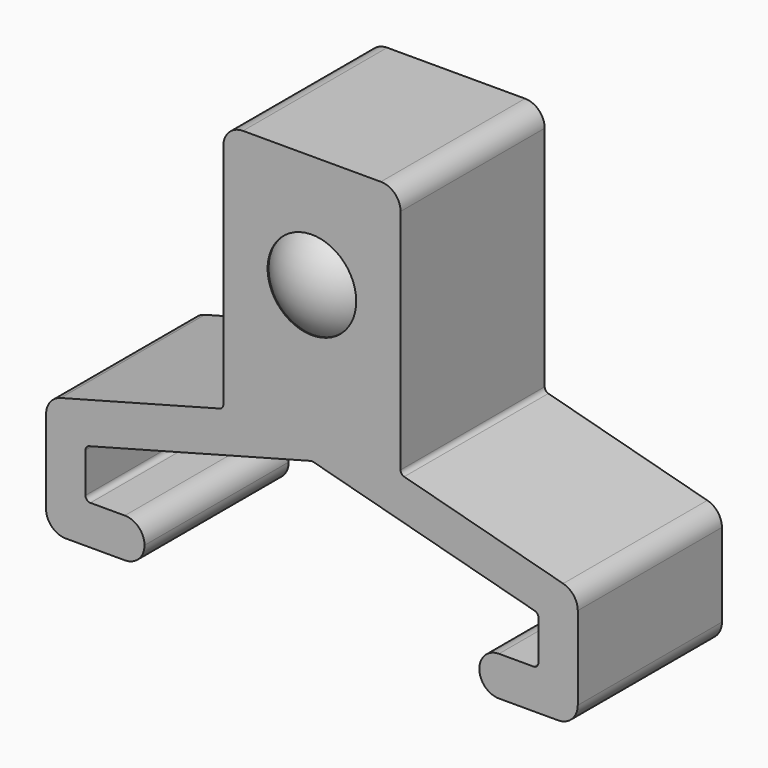
from build123d import *

# Parameters (mm, degrees)
F1_DEPTH      = 4.575
F1_DEPTH_BACK = 4.575
F2_R          = 2.25
F3_DEPTH      = 6
F4_R          = 0.99999
F5_R          = 0.25


# Not quite as in the source:
# - a fillet or chamfer is up to 0.001 mm smaller than in the source, because OpenCascade refuses the exact size


with BuildPart() as f1:
    # F0 (on Front) → F1 (new body, two sides)
    with BuildSketch(Plane.XZ) as f1_sk:
        Polygon((-13.5, 3), (-13.5, -3), (-8.5, -3), (-8.5, -1), (-11.5, -1), (-11.5, 1.4634433738), (0, 4.5301100405), (11.5, 1.4634433738), (11.5, -1), (8.5, -1), (8.5, -3), (13.5, -3), (13.5, 3), (4.5, 5.4), (4.5, 18.15), (-4.5, 18.15), (-4.5, 5.4), align=None)
    extrude(amount=F1_DEPTH)
    extrude(f1_sk.sketch, amount=-F1_DEPTH_BACK)

    # F2 (on face) → F3 (cut)
    with BuildSketch(Plane.XZ.offset(4.575)):
        with Locations((0, 12.4)):
            Circle(F2_R)
    extrude(amount=-F3_DEPTH, mode=Mode.SUBTRACT)

    # F4 (radius 1 in the source; OpenCascade refuses exactly that, so slightly less here)
    f4_edges = [f1.edges().sort_by_distance(p)[0] for p in [
        (-4.5, 0, 18.15),
        (4.5, 0, 18.15),
        (13.5, 0, 3),
        (13.5, 0, -3),
        (8.5, 0, -3),
        (8.5, 0, -1),
        (-8.5, 0, -3),
        (-8.5, 0, -1),
        (-13.5, 0, 3),
        (-13.5, 0, -3),
    ]]
    fillet(f4_edges, radius=F4_R)

    # F5
    f5_edges = [f1.edges().sort_by_distance(p)[0] for p in [
        (4.5, 0, 5.4),
        (-11.5, 0, -1),
        (-11.5, 0, 1.463443),
        (11.5, 0, -1),
        (11.5, 0, 1.463443),
        (0, 0, 4.53011),
        (-4.5, 0, 5.4),
    ]]
    fillet(f5_edges, radius=F5_R)


with BuildPart() as f8:
    # F7 (on offset) → F8 (revolve)
    with BuildSketch(Plane.XZ.offset(2.55)):
        with BuildLine():
            Line((0, 15.4), (0, 9.4))
            ThreePointArc((0, 9.4), (3, 12.4), (0, 15.4))
        make_face()
    revolve(axis=Axis((0, -2.55, 12.4), (0, 0, -1)))


solid = Compound([f1.part, f8.part])
